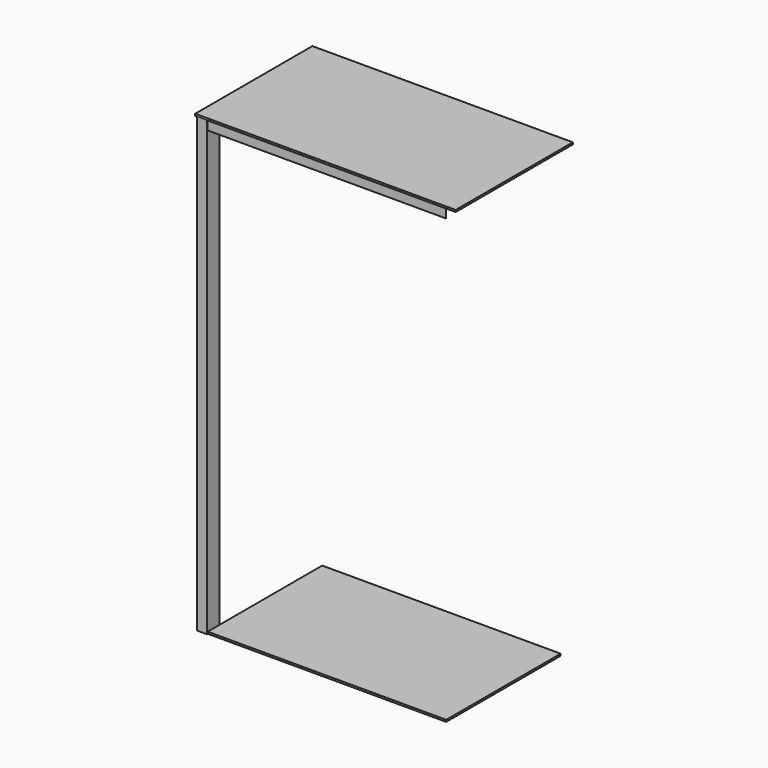
from build123d import *

# Parameters (mm, degrees)
F0_W      = 21
F0_H      = 33
F1_DEPTH  = 950
F3_W      = 12
F3_H      = 21
F4_DEPTH  = 300
F5_SIZE   = 11.99999
F6_W      = 12
F6_H      = 21
F7_DEPTH  = 500
F8_SIZE   = 11.99999
F9_W      = 546
F9_H      = 307
F10_DEPTH = 4
F11_W     = 500
F11_H     = 300
F12_DEPTH = 4


# Not quite as in the source:
# - a fillet or chamfer is up to 0.001 mm smaller than in the source, because OpenCascade refuses the exact size


with BuildPart() as f1:
    # F0 (on Top) → F1 (new body)
    with BuildSketch(Plane.XY):
        with Locations((10.5, 16.5)):
            Rectangle(F0_W, F0_H)
    extrude(amount=F1_DEPTH)


with BuildPart() as f4:
    # F3 (on offset) → F4 (new body)
    with BuildSketch(Plane.XZ.offset(-2)):
        with Locations((27, 939.5)):
            Rectangle(F3_W, F3_H)
    extrude(amount=-F4_DEPTH)

    # F5 (size 12 in the source; OpenCascade refuses exactly that, so slightly less here)
    f5_edges = [f4.edges().sort_by_distance(p)[0] for p in [
        (33, 2, 939.5),
        (33, 302, 939.5),
    ]]
    chamfer(f5_edges, length=F5_SIZE)


with BuildPart() as f7:
    # F6 (on face) → F7 (new body)
    with BuildSketch(Plane.YZ.offset(21)):
        with Locations((8, 939.5)):
            Rectangle(F6_W, F6_H)
    extrude(amount=F7_DEPTH)

    # F8 (size 12 in the source; OpenCascade refuses exactly that, so slightly less here)
    f8_edges = [f7.edges().sort_by_distance(p)[0] for p in [
        (21, 14, 939.5),
        (521, 14, 939.5),
    ]]
    chamfer(f8_edges, length=F8_SIZE)


with BuildPart() as f10:
    # F9 (on face) → F10 (new body)
    with BuildSketch(Plane.XY.offset(950)):
        with Locations((271, 151.5)):
            Rectangle(F9_W, F9_H)
    extrude(amount=F10_DEPTH)


with BuildPart() as f12:
    # F11 (on Top) → F12 (new body)
    with BuildSketch(Plane.XY):
        with Locations((271, 152)):
            Rectangle(F11_W, F11_H)
    extrude(amount=F12_DEPTH)


solid = Compound([f1.part, f4.part, f7.part, f10.part, f12.part])
